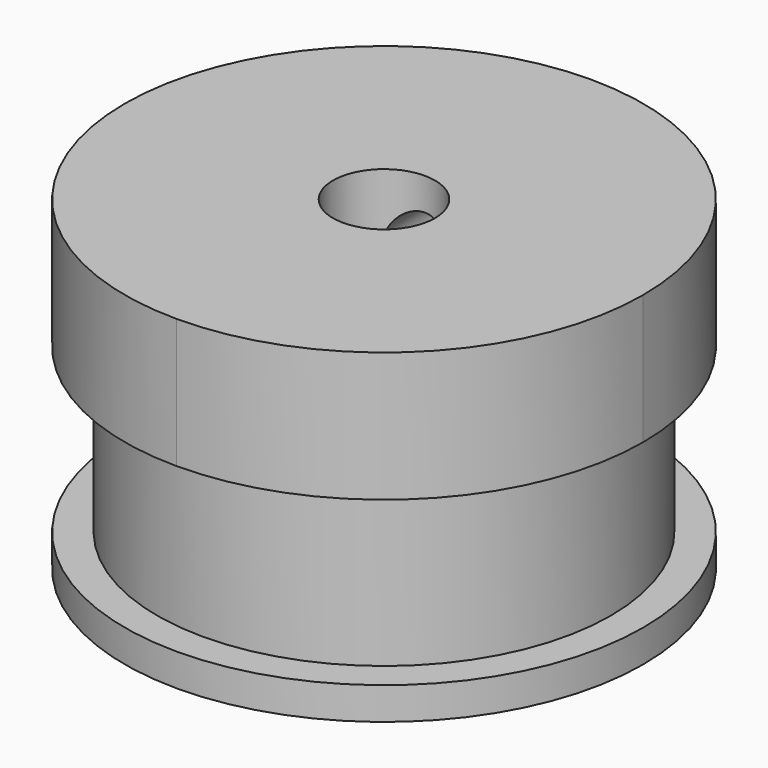
from build123d import *

# Parameters (mm, degrees)
F0_R         = 12.7
F1_DEPTH     = 1.5875
F2_R         = 11.1125
F3_DEPTH     = 8
F4_W         = 25.4
F4_H         = 25.4
F5_DEPTH     = 6.35
F6_R         = 2.5
F7_DEPTH     = 15.9375
F8_R         = 1.5875
F9_REACH     = 29.8911280605
F10_T1_DEPTH = 69.85


# Not quite as in the source:
# - a fillet or chamfer that OpenCascade refuses, or shapes differently, is made with other operations: its cross-section is extruded or revolved along the edge and cut away or added


with BuildPart() as f1:
    # F0 (on Top) → F1 (new body)
    with BuildSketch(Plane.XY):
        Circle(F0_R)
    extrude(amount=F1_DEPTH)

    # F2 (on face) → F3 (join)
    with BuildSketch(Plane.XY.offset(1.5875)):
        Circle(F2_R)
    extrude(amount=F3_DEPTH)

    # F4 (on face) → F5 (join)
    with BuildSketch(Plane.XY.offset(9.5875)):
        Rectangle(F4_W, F4_H)
    extrude(amount=F5_DEPTH)

    # F6 (on face) → F7 (cut, through all)
    with BuildSketch(Plane.XY.offset(15.9375)):
        Circle(F6_R)
    extrude(amount=-F7_DEPTH, mode=Mode.SUBTRACT)

    f9_end = f1.faces().sort_by_distance((-2.5, 0, 7.96875))[0]
    # F8 (on face) → F9 (cut, up to a face of the model that its end follows)
    with BuildSketch(Plane(origin=(0, 12.7, 0), x_dir=(-1, 0, 0), z_dir=(0, 1, 0))):
        with Locations((0, 12.7625)):
            Circle(F8_R)
    f9_long = extrude(amount=-F9_REACH, mode=Mode.PRIVATE)
    add(split(f9_long, bisect_by=f9_end, keep=Keep.ALL, mode=Mode.PRIVATE).solids().sort_by_distance((0, 12.7, 12.7625))[0], mode=Mode.SUBTRACT)

    # F10: fillet of radius 12.7 on 4 edges, made by hand

    # F10_s2 → F10_t1 (cut)
    with BuildSketch(Plane.XY.offset(-22.1625)):
        with BuildLine():
            ThreePointArc((-12.7, 0), (-8.9802561211, 8.9802561211), (0, 12.7))
            Line((0, 12.7), (-12.7, 12.7))
            Line((-12.7, 12.7), (-12.7, 0))
        make_face()
        with BuildLine():
            ThreePointArc((0, -12.7), (-8.9802561211, -8.9802561211), (-12.7, 0))
            Line((-12.7, 0), (-12.7, -12.7))
            Line((-12.7, -12.7), (0, -12.7))
        make_face()
        with BuildLine():
            ThreePointArc((12.7, 0), (8.9802561211, 8.9802561211), (0, 12.7))
            Line((0, 12.7), (12.7, 12.7))
            Line((12.7, 12.7), (12.7, 0))
        make_face()
        with BuildLine():
            ThreePointArc((0, -12.7), (8.9802561211, -8.9802561211), (12.7, 0))
            Line((12.7, 0), (12.7, -12.7))
            Line((12.7, -12.7), (0, -12.7))
        make_face()
    extrude(amount=F10_T1_DEPTH, mode=Mode.SUBTRACT)


solid = f1.part
